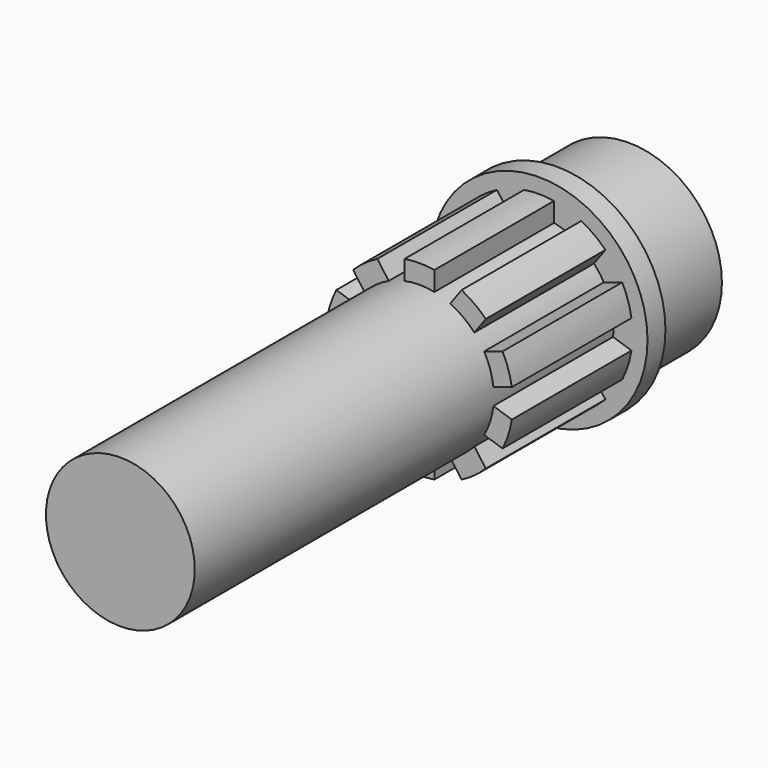
from build123d import *

# Parameters (mm, degrees)
F0_R     = 12.45
F1_DEPTH = 12
F2_R     = 14.5
F3_DEPTH = 3
F4_R     = 9.95
F5_DEPTH = 70
F7_DEPTH = 20


with BuildPart() as f1:
    # F0 (on Front) → F1 (new body)
    with BuildSketch(Plane.XZ):
        Circle(F0_R)
    extrude(amount=F1_DEPTH)

    # F2 (on face) → F3 (join)
    with BuildSketch(Plane.XZ.offset(12)):
        Circle(F2_R)
    extrude(amount=F3_DEPTH)

    # F4 (on face) → F5 (join)
    with BuildSketch(Plane.XZ.offset(15)):
        Circle(F4_R)
    extrude(amount=F5_DEPTH)

    # F6 (on face) → F7 (join)
    with BuildSketch(Plane.XZ.offset(15)):
        with BuildLine():
            Line((2, 9.7469225913), (2, 12.3389626793))
            ThreePointArc((2, 12.3389626793), (0, 12.5), (-2, 12.3389626793))
            Line((-2, 12.3389626793), (-2, 9.7469225913))
            ThreePointArc((-2, 9.7469225913), (0, 9.95), (2, 9.7469225913))
        make_face()
        with BuildLine():
            ThreePointArc((-7.3471313431, 6.7098555146), (-5.8484632603, 8.049719094), (-4.1110633656, 9.0609965238))
            Line((-4.1110633656, 9.0609965238), (-5.6346263027, 11.1580010051))
            ThreePointArc((-5.6346263027, 11.1580010051), (-7.3473156537, 10.1127124297), (-8.8706942802, 8.8068599959))
            Line((-8.8706942802, 8.8068599959), (-7.3471313431, 6.7098555146))
        make_face()
        with BuildLine():
            ThreePointArc((-9.887908233, 1.109851691), (-9.4630123371, 3.074719094), (-8.6518402555, 4.9140777561))
            Line((-8.6518402555, 4.9140777561), (-11.1170168717, 5.7150621934))
            ThreePointArc((-11.1170168717, 5.7150621934), (-11.8882064537, 3.8627124297), (-12.3530848492, 1.9108361283))
            Line((-12.3530848492, 1.9108361283), (-9.887908233, 1.109851691))
        make_face()
        with BuildLine():
            ThreePointArc((-8.6518402555, -4.9140777561), (-9.4630123371, -3.074719094), (-9.887908233, -1.109851691))
            Line((-9.887908233, -1.109851691), (-12.3530848492, -1.9108361283))
            ThreePointArc((-12.3530848492, -1.9108361283), (-11.8882064537, -3.8627124297), (-11.1170168717, -5.7150621934))
            Line((-11.1170168717, -5.7150621934), (-8.6518402555, -4.9140777561))
        make_face()
        with BuildLine():
            ThreePointArc((-4.1110633656, -9.0609965238), (-5.8484632603, -8.049719094), (-7.3471313431, -6.7098555146))
            Line((-7.3471313431, -6.7098555146), (-8.8706942802, -8.8068599959))
            ThreePointArc((-8.8706942802, -8.8068599959), (-7.3473156537, -10.1127124297), (-5.6346263027, -11.1580010051))
            Line((-5.6346263027, -11.1580010051), (-4.1110633656, -9.0609965238))
        make_face()
        with BuildLine():
            ThreePointArc((2, -9.7469225913), (0, -9.95), (-2, -9.7469225913))
            Line((-2, -9.7469225913), (-2, -12.3389626793))
            ThreePointArc((-2, -12.3389626793), (0, -12.5), (2, -12.3389626793))
            Line((2, -12.3389626793), (2, -9.7469225913))
        make_face()
        with BuildLine():
            Line((8.8706942802, -8.8068599959), (7.3471313431, -6.7098555146))
            ThreePointArc((7.3471313431, -6.7098555146), (5.8484632603, -8.049719094), (4.1110633656, -9.0609965238))
            Line((4.1110633656, -9.0609965238), (5.6346263027, -11.1580010051))
            ThreePointArc((5.6346263027, -11.1580010051), (7.3473156537, -10.1127124297), (8.8706942802, -8.8068599959))
        make_face()
        with BuildLine():
            Line((12.3530848492, -1.9108361283), (9.887908233, -1.109851691))
            ThreePointArc((9.887908233, -1.109851691), (9.4630123371, -3.074719094), (8.6518402555, -4.9140777561))
            Line((8.6518402555, -4.9140777561), (11.1170168717, -5.7150621934))
            ThreePointArc((11.1170168717, -5.7150621934), (11.8882064537, -3.8627124297), (12.3530848492, -1.9108361283))
        make_face()
        with BuildLine():
            Line((11.1170168717, 5.7150621934), (8.6518402555, 4.9140777561))
            ThreePointArc((8.6518402555, 4.9140777561), (9.4630123371, 3.074719094), (9.887908233, 1.109851691))
            Line((9.887908233, 1.109851691), (12.3530848492, 1.9108361283))
            ThreePointArc((12.3530848492, 1.9108361283), (11.8882064537, 3.8627124297), (11.1170168717, 5.7150621934))
        make_face()
        with BuildLine():
            Line((5.6346263027, 11.1580010051), (4.1110633656, 9.0609965238))
            ThreePointArc((4.1110633656, 9.0609965238), (5.8484632603, 8.049719094), (7.3471313431, 6.7098555146))
            Line((7.3471313431, 6.7098555146), (8.8706942802, 8.8068599959))
            ThreePointArc((8.8706942802, 8.8068599959), (7.3473156537, 10.1127124297), (5.6346263027, 11.1580010051))
        make_face()
    extrude(amount=F7_DEPTH)


solid = f1.part
